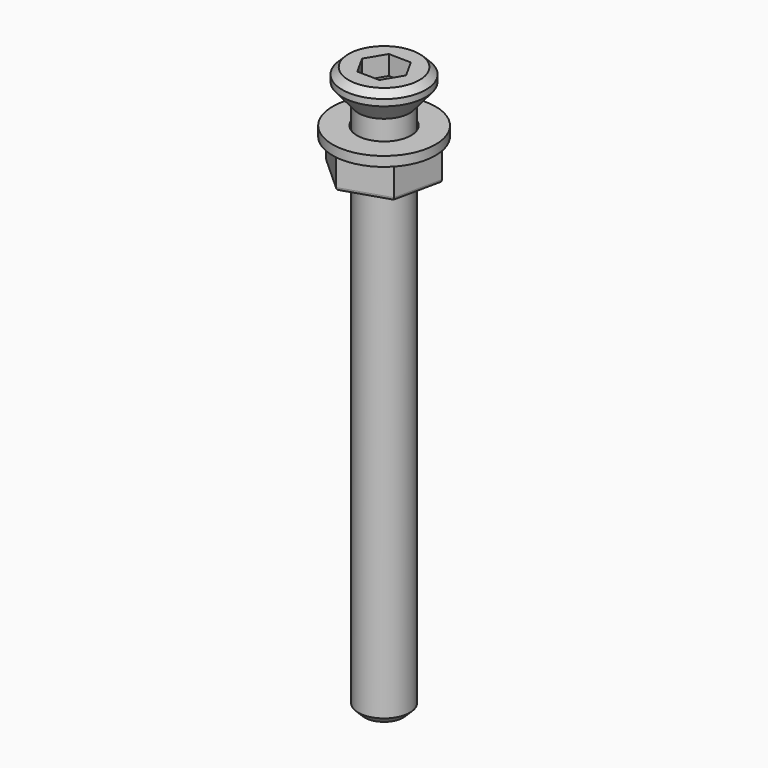
from build123d import *

# Parameters (mm, degrees)
F0_R         = 6.5
F1_DEPTH     = 8
F2_R         = 4
F3_DEPTH     = 80
F5_DEPTH     = 3
F6_SIZE      = 1
F7_R         = 4
F8_DEPTH     = 6.5
F9_R         = 0.5
F10_R        = 8
F10_R_2      = 4.2
F11_DEPTH    = 1.5
F12_S5_R     = 4
F12_T6_DEPTH = 11


# Not quite as in the source:
# - a fillet or chamfer that OpenCascade refuses, or shapes differently, is made with other operations: its cross-section is extruded or revolved along the edge and cut away or added


with BuildPart() as f1:
    # F0 (on Top) → F1 (new body)
    with BuildSketch(Plane.XY):
        Circle(F0_R)
    extrude(amount=F1_DEPTH)

    # F2 (on face) → F3 (join)
    with BuildSketch(Plane(origin=(0, 0, 0), x_dir=(1, 0, 0), z_dir=(0, 0, -1))):
        Circle(F2_R)
    extrude(amount=F3_DEPTH)

    # F4 (on face) → F5 (cut)
    with BuildSketch(Plane.XY.offset(8)):
        Polygon((-1.6792826051, 3.0298531206), (-3.4635710747, 0.0606251641), (-1.7842884696, -2.9692279564), (1.6792826051, -3.0298531206), (3.4635710747, -0.0606251641), (1.7842884696, 2.9692279564), align=None)
    extrude(amount=-F5_DEPTH, mode=Mode.SUBTRACT)

    # F6
    f6_edges = [f1.edges().sort_by_distance(p)[0] for p in [
        (-4, 0, -80),
        (-6.5, 0, 8),
    ]]
    chamfer(f6_edges, length=F6_SIZE)

    # F12: chamfer of 6 x 5 on 1 edges, made by hand


with BuildPart() as f8:
    # F7 (on face) → F8 (new body)
    with BuildSketch(Plane(origin=(0, 0, 0), x_dir=(1, 0, 0), z_dir=(0, 0, -1))):
        Polygon((1.5766953018, -7.3380764004), (7.1433082286, -2.3035800149), (5.5666129268, 5.0344963856), (-1.5766953018, 7.3380764004), (-7.1433082286, 2.3035800149), (-5.5666129268, -5.0344963856), align=None)
        Circle(F7_R, mode=Mode.SUBTRACT)
    extrude(amount=F8_DEPTH)

    # F9
    f9_edges = [f8.edges().sort_by_distance(p)[0] for p in [
        (-6.354961, 1.365458, -6.5),
        (-1.994959, 6.186286, -6.5),
        (4.360002, 4.820828, -6.5),
        (6.354961, -1.365458, -6.5),
        (1.994959, -6.186286, -6.5),
        (-4.360002, -4.820828, -6.5),
        (-4, 0, -6.5),
        (-6.354961, 1.365458, 0),
        (-1.994959, 6.186286, 0),
        (4.360002, 4.820828, 0),
        (6.354961, -1.365458, 0),
        (1.994959, -6.186286, 0),
        (-4.360002, -4.820828, 0),
        (-4, 0, 0),
    ]]
    fillet(f9_edges, radius=F9_R)


with BuildPart() as f11:
    # F10 (on face) → F11 (new body)
    with BuildSketch(Plane(origin=(0, 0, 0), x_dir=(1, 0, 0), z_dir=(0, 0, -1))):
        Circle(F10_R)
        Circle(F10_R_2, mode=Mode.SUBTRACT)
    extrude(amount=F11_DEPTH)


with BuildPart() as f12_tool2:
    # F12_s3 → F12_t4 (revolve)
    with BuildSketch(Plane.XZ):
        Polygon((6.5, 6), (1.5, 0), (6.5, 0), align=None)
    revolve(axis=Axis((0, 0, 0), (0, 0, 1)))

    # F12_s5 → F12_t6 (cut, symmetric)
    with BuildSketch(Plane.XY.offset(3)):
        Circle(F12_S5_R)
    extrude(amount=F12_T6_DEPTH, both=True, mode=Mode.SUBTRACT)


with BuildPart() as f1_1:
    add(f1.part)

    # F12_t1: cut F12_tool2
    add(f12_tool2.part, mode=Mode.SUBTRACT)


solid = Compound([f8.part, f11.part, f1_1.part])
